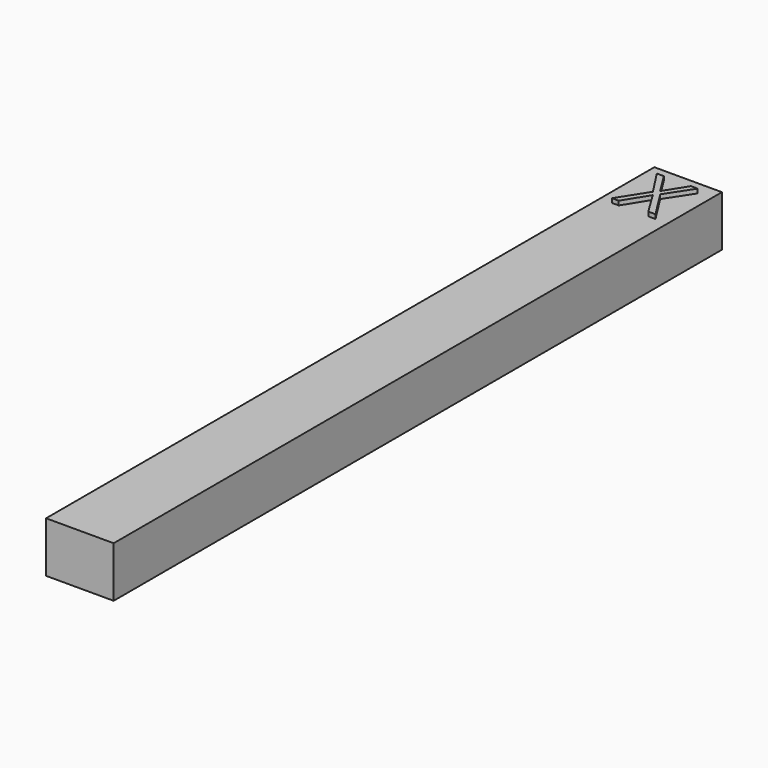
from build123d import *

# Parameters (mm, degrees)
F0_W         = 8
F0_H         = 6
F1_DEPTH     = 90
F2_TEXT_SIZE = 9.0267966799
F3_DEPTH     = 0.5


# Not quite as in the source:
# - Text() gives the source's letters only with a copy of the font that has no kerning and outlines rounded to 1/6400 em; it was checked with that copy


with BuildPart() as f1:
    # F0 (on Front) → F1 (new body)
    with BuildSketch(Plane.XZ):
        Rectangle(F0_W, F0_H)
    extrude(amount=F1_DEPTH)

    # F2 (on face) → F3 (join)
    with BuildSketch(Plane.XY.offset(3)):
        with Locations((-2.6102457196, -8.0401180312)):
            Text('X', F2_TEXT_SIZE, font='Open Sans', text_align=(TextAlign.LEFT, TextAlign.BOTTOM))
    extrude(amount=F3_DEPTH)


solid = f1.part
